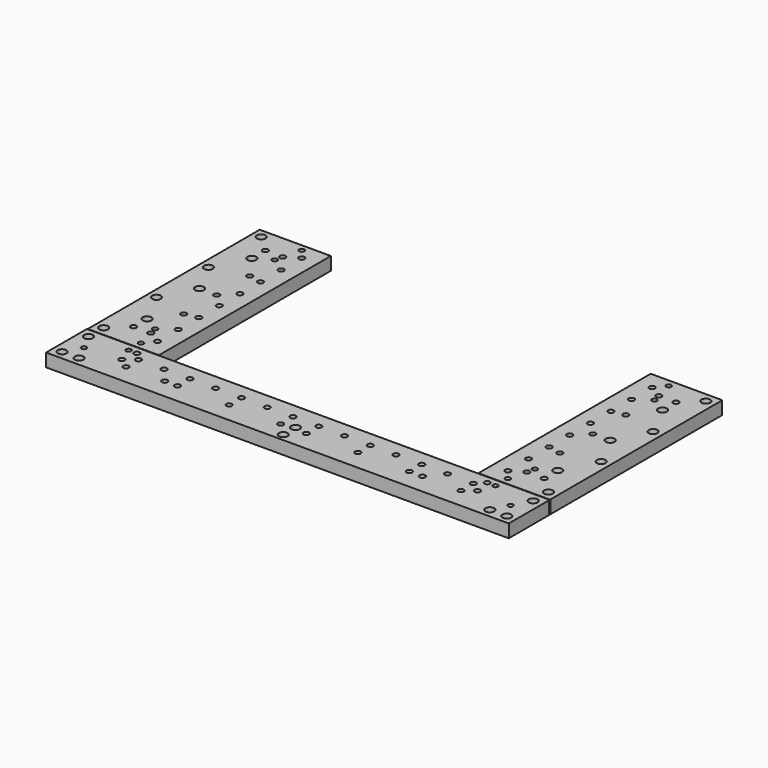
from build123d import *

# Parameters (mm, degrees)
F1_DEPTH = 25.4


# Not quite as in the source:
# - ends of sketch curves that miss each other by under 0.0002 mm in the source are joined


with BuildPart() as f1:
    # F0 (on Top) → F1 (new body)
    with BuildSketch(Plane.XY):
        Polygon((-339.0000078, 258.5000164), (-448.0000184, 258.5000164), (-448.0000184, -157.4999898), (-448.0000184, -158.4999878), (-339.414231, -158.4999878), (-310.000015, -158.4999878), (-310.000015, -157.9999888), (-310.000015, -157.4999898), (-310.000015, 258.5000164), (-310.500014, 258.5000164), align=None)
        with BuildLine():
            ThreePointArc((-431.500026, -149.0000068), (-440.0000344, -140.4999984), (-431.500026, -131.99999))
            ThreePointArc((-431.500026, -131.99999), (-423.0000176, -140.4999984), (-431.500026, -149.0000068))
        make_face(mode=Mode.SUBTRACT)
        with BuildLine():
            ThreePointArc((-356.0000246, -149.4999804), (-361.0000146, -144.4999904), (-356.0000246, -139.5000004))
            ThreePointArc((-356.0000246, -139.5000004), (-351.0000346, -144.4999904), (-356.0000246, -149.4999804))
        make_face(mode=Mode.SUBTRACT)
        with BuildLine():
            ThreePointArc((-398.5000158, -114.9999732), (-404.0000048, -109.4999842), (-398.5000158, -103.9999952))
            ThreePointArc((-398.5000158, -103.9999952), (-393.0000268, -109.4999842), (-398.5000158, -114.9999732))
        make_face(mode=Mode.SUBTRACT)
        with BuildLine():
            ThreePointArc((-340.0000058, -129.999994), (-345.4999948, -124.500005), (-340.0000058, -119.000016))
            ThreePointArc((-340.0000058, -119.000016), (-334.5000168, -124.500005), (-340.0000058, -129.999994))
        make_face(mode=Mode.SUBTRACT)
        with BuildLine():
            ThreePointArc((-365.0000066, -114.9999732), (-370.4999956, -109.4999842), (-365.0000066, -103.9999952))
            ThreePointArc((-365.0000066, -103.9999952), (-359.5000176, -109.4999842), (-365.0000066, -114.9999732))
        make_face(mode=Mode.SUBTRACT)
        with BuildLine():
            ThreePointArc((-398.5000158, -85.0000078), (-407.0000242, -76.4999994), (-398.5000158, -67.999991))
            ThreePointArc((-398.5000158, -67.999991), (-390.0000074, -76.4999994), (-398.5000158, -85.0000078))
        make_face(mode=Mode.SUBTRACT)
        with BuildLine():
            ThreePointArc((-368.500025, -99.4999788), (-373.500015, -94.4999888), (-368.500025, -89.4999988))
            ThreePointArc((-368.500025, -89.4999988), (-363.500035, -94.4999888), (-368.500025, -99.4999788))
        make_face(mode=Mode.SUBTRACT)
        with BuildLine():
            ThreePointArc((-340.0000058, -79.9999924), (-345.4999948, -74.5000034), (-340.0000058, -69.0000144))
            ThreePointArc((-340.0000058, -69.0000144), (-334.5000168, -74.5000034), (-340.0000058, -79.9999924))
        make_face(mode=Mode.SUBTRACT)
        with BuildLine():
            ThreePointArc((-431.500026, -21.0000088), (-440.0000344, -12.5000004), (-431.500026, -3.999992))
            ThreePointArc((-431.500026, -3.999992), (-423.0000176, -12.5000004), (-431.500026, -21.0000088))
        make_face(mode=Mode.SUBTRACT)
        with BuildLine():
            ThreePointArc((-365.0000066, -34.9999808), (-370.4999956, -29.4999918), (-365.0000066, -24.0000028))
            ThreePointArc((-365.0000066, -24.0000028), (-359.5000176, -29.4999918), (-365.0000066, -34.9999808))
        make_face(mode=Mode.SUBTRACT)
        with BuildLine():
            ThreePointArc((-340.0000058, -29.9999908), (-345.4999948, -24.5000018), (-340.0000058, -19.0000128))
            ThreePointArc((-340.0000058, -19.0000128), (-334.5000168, -24.5000018), (-340.0000058, -29.9999908))
        make_face(mode=Mode.SUBTRACT)
        with BuildLine():
            ThreePointArc((-340.0000058, 20.0000108), (-345.4999948, 25.4999998), (-340.0000058, 30.9999888))
            ThreePointArc((-340.0000058, 30.9999888), (-334.5000168, 25.4999998), (-340.0000058, 20.0000108))
        make_face(mode=Mode.SUBTRACT)
        with BuildLine():
            ThreePointArc((-398.5000158, 41.9999922), (-407.0000242, 50.5000006), (-398.5000158, 59.000009))
            ThreePointArc((-398.5000158, 59.000009), (-390.0000074, 50.5000006), (-398.5000158, 41.9999922))
        make_face(mode=Mode.SUBTRACT)
        with BuildLine():
            ThreePointArc((-365.0000066, 45.0000116), (-370.4999956, 50.5000006), (-365.0000066, 55.9999896))
            ThreePointArc((-365.0000066, 55.9999896), (-359.5000176, 50.5000006), (-365.0000066, 45.0000116))
        make_face(mode=Mode.SUBTRACT)
        with BuildLine():
            ThreePointArc((-340.0000058, 70.0000124), (-345.4999948, 75.5000014), (-340.0000058, 80.9999904))
            ThreePointArc((-340.0000058, 80.9999904), (-334.5000168, 75.5000014), (-340.0000058, 70.0000124))
        make_face(mode=Mode.SUBTRACT)
        with BuildLine():
            ThreePointArc((-431.500026, 104.9999932), (-440.0000344, 113.5000016), (-431.500026, 122.00001))
            ThreePointArc((-431.500026, 122.00001), (-423.0000176, 113.5000016), (-431.500026, 104.9999932))
        make_face(mode=Mode.SUBTRACT)
        with BuildLine():
            ThreePointArc((-340.0000058, 120.000014), (-345.4999948, 125.500003), (-340.0000058, 130.999992))
            ThreePointArc((-340.0000058, 130.999992), (-334.5000168, 125.500003), (-340.0000058, 120.000014))
        make_face(mode=Mode.SUBTRACT)
        with BuildLine():
            ThreePointArc((-365.0000066, 125.0000294), (-370.4999956, 130.5000184), (-365.0000066, 136.0000074))
            ThreePointArc((-365.0000066, 136.0000074), (-359.5000176, 130.5000184), (-365.0000066, 125.0000294))
        make_face(mode=Mode.SUBTRACT)
        with BuildLine():
            ThreePointArc((-398.5000158, 168.9999922), (-407.0000242, 177.5000006), (-398.5000158, 186.000009))
            ThreePointArc((-398.5000158, 186.000009), (-390.0000074, 177.5000006), (-398.5000158, 168.9999922))
        make_face(mode=Mode.SUBTRACT)
        with BuildLine():
            ThreePointArc((-340.0000058, 170.0000156), (-345.4999948, 175.5000046), (-340.0000058, 180.9999936))
            ThreePointArc((-340.0000058, 180.9999936), (-334.5000168, 175.5000046), (-340.0000058, 170.0000156))
        make_face(mode=Mode.SUBTRACT)
        with BuildLine():
            ThreePointArc((-398.5000158, 205.0000218), (-404.0000048, 210.5000108), (-398.5000158, 215.9999998))
            ThreePointArc((-398.5000158, 215.9999998), (-393.0000268, 210.5000108), (-398.5000158, 205.0000218))
        make_face(mode=Mode.SUBTRACT)
        with BuildLine():
            ThreePointArc((-368.500025, 190.5000254), (-373.500015, 195.5000154), (-368.500025, 200.5000054))
            ThreePointArc((-368.500025, 200.5000054), (-363.500035, 195.5000154), (-368.500025, 190.5000254))
        make_face(mode=Mode.SUBTRACT)
        with BuildLine():
            ThreePointArc((-365.0000066, 205.0000218), (-370.4999956, 210.5000108), (-365.0000066, 215.9999998))
            ThreePointArc((-365.0000066, 215.9999998), (-359.5000176, 210.5000108), (-365.0000066, 205.0000218))
        make_face(mode=Mode.SUBTRACT)
        with BuildLine():
            ThreePointArc((-340.0000058, 220.0000172), (-345.4999948, 225.5000062), (-340.0000058, 230.9999952))
            ThreePointArc((-340.0000058, 230.9999952), (-334.5000168, 225.5000062), (-340.0000058, 220.0000172))
        make_face(mode=Mode.SUBTRACT)
        with BuildLine():
            ThreePointArc((-431.500026, 232.9999912), (-440.0000344, 241.4999996), (-431.500026, 250.000008))
            ThreePointArc((-431.500026, 250.000008), (-423.0000176, 241.4999996), (-431.500026, 232.9999912))
        make_face(mode=Mode.SUBTRACT)
        with BuildLine():
            ThreePointArc((-356.0000246, 240.500027), (-361.0000146, 245.500017), (-356.0000246, 250.500007))
            ThreePointArc((-356.0000246, 250.500007), (-351.0000346, 245.500017), (-356.0000246, 240.500027))
        make_face(mode=Mode.SUBTRACT)
    extrude(amount=F1_DEPTH)


with BuildPart() as f1b:
    # F0 (on Top) → F1, piece 2 (new body)
    with BuildSketch(Plane.XY):
        Polygon((-448.0000184, -258.499991), (-333.0000198, -258.499991), (-65.0000224, -258.499991), (64.9999716, -258.499991), (332.9999944, -258.499991), (447.999993, -258.499991), (448.999991, -258.499991), (448.999991, -160.4999838), (448.499992, -159.9999848), (447.999993, -159.4999858), (332.9999944, -159.4999858), (-333.0000198, -159.4999858), (-448.0000184, -159.4999858), (-448.2500179, -159.7499853), (-448.5000174, -159.9999848), (-449.0000164, -160.4999838), (-449.0000164, -258.499991), align=None)
        with BuildLine():
            ThreePointArc((-423.0000176, -241.4999996), (-431.500026, -250.000008), (-440.0000344, -241.4999996))
            ThreePointArc((-440.0000344, -241.4999996), (-431.500026, -232.9999912), (-423.0000176, -241.4999996))
        make_face(mode=Mode.SUBTRACT)
        with BuildLine():
            ThreePointArc((-390.0000074, -241.4999996), (-398.5000158, -250.000008), (-407.0000242, -241.4999996))
            ThreePointArc((-407.0000242, -241.4999996), (-398.5000158, -232.9999912), (-390.0000074, -241.4999996))
        make_face(mode=Mode.SUBTRACT)
        with BuildLine():
            ThreePointArc((-409.0000202, -210.4999854), (-414.0000102, -215.4999754), (-419.0000002, -210.4999854))
            ThreePointArc((-419.0000002, -210.4999854), (-414.0000102, -205.4999954), (-409.0000202, -210.4999854))
        make_face(mode=Mode.SUBTRACT)
        with BuildLine():
            ThreePointArc((-339.5000322, -204.4999974), (-345.0000212, -209.9999864), (-350.5000102, -204.4999974))
            ThreePointArc((-350.5000102, -204.4999974), (-345.0000212, -199.0000084), (-339.5000322, -204.4999974))
        make_face(mode=Mode.SUBTRACT)
        with BuildLine():
            ThreePointArc((-319.5000214, -219.4999928), (-325.0000104, -224.9999818), (-330.4999994, -219.4999928))
            ThreePointArc((-330.4999994, -219.4999928), (-325.0000104, -214.0000038), (-319.5000214, -219.4999928))
        make_face(mode=Mode.SUBTRACT)
        with BuildLine():
            ThreePointArc((-244.500019, -219.4999928), (-250.000008, -224.9999818), (-255.499997, -219.4999928))
            ThreePointArc((-255.499997, -219.4999928), (-250.000008, -214.0000038), (-244.500019, -219.4999928))
        make_face(mode=Mode.SUBTRACT)
        with BuildLine():
            ThreePointArc((-219.5000182, -219.4999928), (-225.0000072, -224.9999818), (-230.4999962, -219.4999928))
            ThreePointArc((-230.4999962, -219.4999928), (-225.0000072, -214.0000038), (-219.5000182, -219.4999928))
        make_face(mode=Mode.SUBTRACT)
        with BuildLine():
            ThreePointArc((-423.0000176, -177.5000006), (-431.500026, -186.000009), (-440.0000344, -177.5000006))
            ThreePointArc((-440.0000344, -177.5000006), (-431.500026, -168.9999922), (-423.0000176, -177.5000006))
        make_face(mode=Mode.SUBTRACT)
        with BuildLine():
            ThreePointArc((-351.0000346, -174.4999812), (-356.0000246, -179.4999712), (-361.0000146, -174.4999812))
            ThreePointArc((-361.0000146, -174.4999812), (-356.0000246, -169.4999912), (-351.0000346, -174.4999812))
        make_face(mode=Mode.SUBTRACT)
        with BuildLine():
            ThreePointArc((-334.5000168, -174.4999812), (-340.0000058, -179.9999702), (-345.4999948, -174.4999812))
            ThreePointArc((-345.4999948, -174.4999812), (-340.0000058, -168.9999922), (-334.5000168, -174.4999812))
        make_face(mode=Mode.SUBTRACT)
        with BuildLine():
            ThreePointArc((-319.5000214, -189.500002), (-325.0000104, -194.999991), (-330.4999994, -189.500002))
            ThreePointArc((-330.4999994, -189.500002), (-325.0000104, -184.000013), (-319.5000214, -189.500002))
        make_face(mode=Mode.SUBTRACT)
        with BuildLine():
            ThreePointArc((-269.5000198, -189.500002), (-275.0000088, -194.999991), (-280.4999978, -189.500002))
            ThreePointArc((-280.4999978, -189.500002), (-275.0000088, -184.000013), (-269.5000198, -189.500002))
        make_face(mode=Mode.SUBTRACT)
        with BuildLine():
            ThreePointArc((-219.5000182, -189.500002), (-225.0000072, -194.999991), (-230.4999962, -189.500002))
            ThreePointArc((-230.4999962, -189.500002), (-225.0000072, -184.000013), (-219.5000182, -189.500002))
        make_face(mode=Mode.SUBTRACT)
        with BuildLine():
            ThreePointArc((-119.500015, -219.4999928), (-125.000004, -224.9999818), (-130.499993, -219.4999928))
            ThreePointArc((-130.499993, -219.4999928), (-125.000004, -214.0000038), (-119.500015, -219.4999928))
        make_face(mode=Mode.SUBTRACT)
        with BuildLine():
            ThreePointArc((8.499983, -244.4999936), (-2.54e-05, -253.000002), (-8.5000338, -244.4999936))
            ThreePointArc((-8.5000338, -244.4999936), (-2.54e-05, -235.9999852), (8.499983, -244.4999936))
        make_face(mode=Mode.SUBTRACT)
        with BuildLine():
            ThreePointArc((-19.5000372, -219.4999928), (-25.0000262, -224.9999818), (-30.5000152, -219.4999928))
            ThreePointArc((-30.5000152, -219.4999928), (-25.0000262, -214.0000038), (-19.5000372, -219.4999928))
        make_face(mode=Mode.SUBTRACT)
        with BuildLine():
            ThreePointArc((8.499983, -214.5000028), (-2.54e-05, -223.0000112), (-8.5000338, -214.5000028))
            ThreePointArc((-8.5000338, -214.5000028), (-2.54e-05, -205.9999944), (8.499983, -214.5000028))
        make_face(mode=Mode.SUBTRACT)
        with BuildLine():
            ThreePointArc((-169.5000166, -189.500002), (-175.0000056, -194.999991), (-180.4999946, -189.500002))
            ThreePointArc((-180.4999946, -189.500002), (-175.0000056, -184.000013), (-169.5000166, -189.500002))
        make_face(mode=Mode.SUBTRACT)
        with BuildLine():
            ThreePointArc((-119.500015, -189.500002), (-125.000004, -194.999991), (-130.499993, -189.500002))
            ThreePointArc((-130.499993, -189.500002), (-125.000004, -184.000013), (-119.500015, -189.500002))
        make_face(mode=Mode.SUBTRACT)
        with BuildLine():
            ThreePointArc((-69.5000388, -189.500002), (-75.0000278, -194.999991), (-80.5000168, -189.500002))
            ThreePointArc((-80.5000168, -189.500002), (-75.0000278, -184.000013), (-69.5000388, -189.500002))
        make_face(mode=Mode.SUBTRACT)
        with BuildLine():
            ThreePointArc((-19.5000372, -189.500002), (-25.0000262, -194.999991), (-30.5000152, -189.500002))
            ThreePointArc((-30.5000152, -189.500002), (-25.0000262, -184.000013), (-19.5000372, -189.500002))
        make_face(mode=Mode.SUBTRACT)
        with BuildLine():
            ThreePointArc((30.4999644, -219.4999928), (24.9999754, -224.9999818), (19.4999864, -219.4999928))
            ThreePointArc((19.4999864, -219.4999928), (24.9999754, -214.0000038), (30.4999644, -219.4999928))
        make_face(mode=Mode.SUBTRACT)
        with BuildLine():
            ThreePointArc((130.4999676, -219.4999928), (124.9999786, -224.9999818), (119.4999896, -219.4999928))
            ThreePointArc((119.4999896, -219.4999928), (124.9999786, -214.0000038), (130.4999676, -219.4999928))
        make_face(mode=Mode.SUBTRACT)
        with BuildLine():
            ThreePointArc((30.4999644, -189.500002), (24.9999754, -194.999991), (19.4999864, -189.500002))
            ThreePointArc((19.4999864, -189.500002), (24.9999754, -184.000013), (30.4999644, -189.500002))
        make_face(mode=Mode.SUBTRACT)
        with BuildLine():
            ThreePointArc((80.499966, -189.500002), (74.999977, -194.999991), (69.499988, -189.500002))
            ThreePointArc((69.499988, -189.500002), (74.999977, -184.000013), (80.499966, -189.500002))
        make_face(mode=Mode.SUBTRACT)
        with BuildLine():
            ThreePointArc((130.4999676, -189.500002), (124.9999786, -194.999991), (119.4999896, -189.500002))
            ThreePointArc((119.4999896, -189.500002), (124.9999786, -184.000013), (130.4999676, -189.500002))
        make_face(mode=Mode.SUBTRACT)
        with BuildLine():
            ThreePointArc((180.4999692, -189.500002), (174.9999802, -194.999991), (169.4999912, -189.500002))
            ThreePointArc((169.4999912, -189.500002), (174.9999802, -184.000013), (180.4999692, -189.500002))
        make_face(mode=Mode.SUBTRACT)
        with BuildLine():
            ThreePointArc((230.4999708, -219.4999928), (224.9999818, -224.9999818), (219.4999928, -219.4999928))
            ThreePointArc((219.4999928, -219.4999928), (224.9999818, -214.0000038), (230.4999708, -219.4999928))
        make_face(mode=Mode.SUBTRACT)
        with BuildLine():
            ThreePointArc((255.4999716, -219.4999928), (249.9999826, -224.9999818), (244.4999936, -219.4999928))
            ThreePointArc((244.4999936, -219.4999928), (249.9999826, -214.0000038), (255.4999716, -219.4999928))
        make_face(mode=Mode.SUBTRACT)
        with BuildLine():
            ThreePointArc((330.499974, -219.4999928), (324.999985, -224.9999818), (319.499996, -219.4999928))
            ThreePointArc((319.499996, -219.4999928), (324.999985, -214.0000038), (330.499974, -219.4999928))
        make_face(mode=Mode.SUBTRACT)
        with BuildLine():
            ThreePointArc((406.9999988, -241.4999996), (398.4999904, -250.000008), (389.999982, -241.4999996))
            ThreePointArc((389.999982, -241.4999996), (398.4999904, -232.9999912), (406.9999988, -241.4999996))
        make_face(mode=Mode.SUBTRACT)
        with BuildLine():
            ThreePointArc((439.9999836, -241.4999996), (431.4999752, -250.000008), (422.9999668, -241.4999996))
            ThreePointArc((422.9999668, -241.4999996), (431.4999752, -232.9999912), (439.9999836, -241.4999996))
        make_face(mode=Mode.SUBTRACT)
        with BuildLine():
            ThreePointArc((350.4999848, -204.4999974), (344.9999958, -209.9999864), (339.5000068, -204.4999974))
            ThreePointArc((339.5000068, -204.4999974), (344.9999958, -199.0000084), (350.4999848, -204.4999974))
        make_face(mode=Mode.SUBTRACT)
        with BuildLine():
            ThreePointArc((418.9999748, -210.4999854), (413.9999848, -215.4999754), (408.9999948, -210.4999854))
            ThreePointArc((408.9999948, -210.4999854), (413.9999848, -205.4999954), (418.9999748, -210.4999854))
        make_face(mode=Mode.SUBTRACT)
        with BuildLine():
            ThreePointArc((230.4999708, -189.500002), (224.9999818, -194.999991), (219.4999928, -189.500002))
            ThreePointArc((219.4999928, -189.500002), (224.9999818, -184.000013), (230.4999708, -189.500002))
        make_face(mode=Mode.SUBTRACT)
        with BuildLine():
            ThreePointArc((280.4999724, -189.500002), (274.9999834, -194.999991), (269.4999944, -189.500002))
            ThreePointArc((269.4999944, -189.500002), (274.9999834, -184.000013), (280.4999724, -189.500002))
        make_face(mode=Mode.SUBTRACT)
        with BuildLine():
            ThreePointArc((330.499974, -189.500002), (324.999985, -194.999991), (319.499996, -189.500002))
            ThreePointArc((319.499996, -189.500002), (324.999985, -184.000013), (330.499974, -189.500002))
        make_face(mode=Mode.SUBTRACT)
        with BuildLine():
            ThreePointArc((345.4999694, -174.4999812), (339.9999804, -179.9999702), (334.4999914, -174.4999812))
            ThreePointArc((334.4999914, -174.4999812), (339.9999804, -168.9999922), (345.4999694, -174.4999812))
        make_face(mode=Mode.SUBTRACT)
        with BuildLine():
            ThreePointArc((360.9999638, -174.4999812), (355.9999738, -179.4999712), (350.9999838, -174.4999812))
            ThreePointArc((350.9999838, -174.4999812), (355.9999738, -169.4999912), (360.9999638, -174.4999812))
        make_face(mode=Mode.SUBTRACT)
        with BuildLine():
            ThreePointArc((439.9999836, -177.5000006), (431.4999752, -186.000009), (422.9999668, -177.5000006))
            ThreePointArc((422.9999668, -177.5000006), (431.4999752, -168.9999922), (439.9999836, -177.5000006))
        make_face(mode=Mode.SUBTRACT)
    extrude(amount=F1_DEPTH)


with BuildPart() as f1c:
    # F0 (on Top) → F1, piece 3 (new body)
    with BuildSketch(Plane.XY):
        Polygon((309.9999896, 258.5000164), (309.9999896, -157.4999898), (309.9999896, -157.9999888), (309.9999896, -158.4999878), (339.4142056, -158.4999878), (447.999993, -158.4999878), (448.499992, -157.9999888), (448.999991, -157.4999898), (448.999991, 258.5000164), (448.499992, 259.0000154), (447.999993, 259.5000144), (339.4142056, 259.5000144), (309.9999896, 259.5000144), (309.9999896, 259.0000154), (310.4999886, 258.5000164), align=None)
        with BuildLine():
            ThreePointArc((355.9999738, -139.5000004), (360.9999638, -144.4999904), (355.9999738, -149.4999804))
            ThreePointArc((355.9999738, -149.4999804), (350.9999838, -144.4999904), (355.9999738, -139.5000004))
        make_face(mode=Mode.SUBTRACT)
        with BuildLine():
            ThreePointArc((431.4999752, -131.99999), (439.9999836, -140.4999984), (431.4999752, -149.0000068))
            ThreePointArc((431.4999752, -149.0000068), (422.9999668, -140.4999984), (431.4999752, -131.99999))
        make_face(mode=Mode.SUBTRACT)
        with BuildLine():
            ThreePointArc((339.9999804, -119.000016), (345.4999694, -124.500005), (339.9999804, -129.999994))
            ThreePointArc((339.9999804, -129.999994), (334.4999914, -124.500005), (339.9999804, -119.000016))
        make_face(mode=Mode.SUBTRACT)
        with BuildLine():
            ThreePointArc((364.9999812, -103.9999952), (370.4999702, -109.4999842), (364.9999812, -114.9999732))
            ThreePointArc((364.9999812, -114.9999732), (359.4999922, -109.4999842), (364.9999812, -103.9999952))
        make_face(mode=Mode.SUBTRACT)
        with BuildLine():
            ThreePointArc((398.4999904, -103.9999952), (403.9999794, -109.4999842), (398.4999904, -114.9999732))
            ThreePointArc((398.4999904, -114.9999732), (393.0000014, -109.4999842), (398.4999904, -103.9999952))
        make_face(mode=Mode.SUBTRACT)
        with BuildLine():
            ThreePointArc((368.4999742, -89.4999988), (373.4999642, -94.4999888), (368.4999742, -99.4999788))
            ThreePointArc((368.4999742, -99.4999788), (363.4999842, -94.4999888), (368.4999742, -89.4999988))
        make_face(mode=Mode.SUBTRACT)
        with BuildLine():
            ThreePointArc((339.9999804, -69.0000144), (345.4999694, -74.5000034), (339.9999804, -79.9999924))
            ThreePointArc((339.9999804, -79.9999924), (334.4999914, -74.5000034), (339.9999804, -69.0000144))
        make_face(mode=Mode.SUBTRACT)
        with BuildLine():
            ThreePointArc((398.4999904, -67.999991), (406.9999988, -76.4999994), (398.4999904, -85.0000078))
            ThreePointArc((398.4999904, -85.0000078), (389.999982, -76.4999994), (398.4999904, -67.999991))
        make_face(mode=Mode.SUBTRACT)
        with BuildLine():
            ThreePointArc((339.9999804, -19.0000128), (345.4999694, -24.5000018), (339.9999804, -29.9999908))
            ThreePointArc((339.9999804, -29.9999908), (334.4999914, -24.5000018), (339.9999804, -19.0000128))
        make_face(mode=Mode.SUBTRACT)
        with BuildLine():
            ThreePointArc((364.9999812, -24.0000028), (370.4999702, -29.4999918), (364.9999812, -34.9999808))
            ThreePointArc((364.9999812, -34.9999808), (359.4999922, -29.4999918), (364.9999812, -24.0000028))
        make_face(mode=Mode.SUBTRACT)
        with BuildLine():
            ThreePointArc((431.4999752, -3.999992), (439.9999836, -12.5000004), (431.4999752, -21.0000088))
            ThreePointArc((431.4999752, -21.0000088), (422.9999668, -12.5000004), (431.4999752, -3.999992))
        make_face(mode=Mode.SUBTRACT)
        with BuildLine():
            ThreePointArc((339.9999804, 30.9999888), (345.4999694, 25.4999998), (339.9999804, 20.0000108))
            ThreePointArc((339.9999804, 20.0000108), (334.4999914, 25.4999998), (339.9999804, 30.9999888))
        make_face(mode=Mode.SUBTRACT)
        with BuildLine():
            ThreePointArc((364.9999812, 55.9999896), (370.4999702, 50.5000006), (364.9999812, 45.0000116))
            ThreePointArc((364.9999812, 45.0000116), (359.4999922, 50.5000006), (364.9999812, 55.9999896))
        make_face(mode=Mode.SUBTRACT)
        with BuildLine():
            ThreePointArc((398.4999904, 59.000009), (406.9999988, 50.5000006), (398.4999904, 41.9999922))
            ThreePointArc((398.4999904, 41.9999922), (389.999982, 50.5000006), (398.4999904, 59.000009))
        make_face(mode=Mode.SUBTRACT)
        with BuildLine():
            ThreePointArc((339.9999804, 80.9999904), (345.4999694, 75.5000014), (339.9999804, 70.0000124))
            ThreePointArc((339.9999804, 70.0000124), (334.4999914, 75.5000014), (339.9999804, 80.9999904))
        make_face(mode=Mode.SUBTRACT)
        with BuildLine():
            ThreePointArc((339.9999804, 130.999992), (345.4999694, 125.500003), (339.9999804, 120.000014))
            ThreePointArc((339.9999804, 120.000014), (334.4999914, 125.500003), (339.9999804, 130.999992))
        make_face(mode=Mode.SUBTRACT)
        with BuildLine():
            ThreePointArc((431.4999752, 122.00001), (439.9999836, 113.5000016), (431.4999752, 104.9999932))
            ThreePointArc((431.4999752, 104.9999932), (422.9999668, 113.5000016), (431.4999752, 122.00001))
        make_face(mode=Mode.SUBTRACT)
        with BuildLine():
            ThreePointArc((364.9999812, 136.0000074), (370.4999702, 130.5000184), (364.9999812, 125.0000294))
            ThreePointArc((364.9999812, 125.0000294), (359.4999922, 130.5000184), (364.9999812, 136.0000074))
        make_face(mode=Mode.SUBTRACT)
        with BuildLine():
            ThreePointArc((339.9999804, 180.9999936), (345.4999694, 175.5000046), (339.9999804, 170.0000156))
            ThreePointArc((339.9999804, 170.0000156), (334.4999914, 175.5000046), (339.9999804, 180.9999936))
        make_face(mode=Mode.SUBTRACT)
        with BuildLine():
            ThreePointArc((398.4999904, 186.000009), (406.9999988, 177.5000006), (398.4999904, 168.9999922))
            ThreePointArc((398.4999904, 168.9999922), (389.999982, 177.5000006), (398.4999904, 186.000009))
        make_face(mode=Mode.SUBTRACT)
        with BuildLine():
            ThreePointArc((368.4999742, 200.5000054), (373.4999642, 195.5000154), (368.4999742, 190.5000254))
            ThreePointArc((368.4999742, 190.5000254), (363.4999842, 195.5000154), (368.4999742, 200.5000054))
        make_face(mode=Mode.SUBTRACT)
        with BuildLine():
            ThreePointArc((364.9999812, 215.9999998), (370.4999702, 210.5000108), (364.9999812, 205.0000218))
            ThreePointArc((364.9999812, 205.0000218), (359.4999922, 210.5000108), (364.9999812, 215.9999998))
        make_face(mode=Mode.SUBTRACT)
        with BuildLine():
            ThreePointArc((339.9999804, 230.9999952), (345.4999694, 225.5000062), (339.9999804, 220.0000172))
            ThreePointArc((339.9999804, 220.0000172), (334.4999914, 225.5000062), (339.9999804, 230.9999952))
        make_face(mode=Mode.SUBTRACT)
        with BuildLine():
            ThreePointArc((398.4999904, 215.9999998), (403.9999794, 210.5000108), (398.4999904, 205.0000218))
            ThreePointArc((398.4999904, 205.0000218), (393.0000014, 210.5000108), (398.4999904, 215.9999998))
        make_face(mode=Mode.SUBTRACT)
        with BuildLine():
            ThreePointArc((355.9999738, 250.500007), (360.9999638, 245.500017), (355.9999738, 240.500027))
            ThreePointArc((355.9999738, 240.500027), (350.9999838, 245.500017), (355.9999738, 250.500007))
        make_face(mode=Mode.SUBTRACT)
        with BuildLine():
            ThreePointArc((431.4999752, 250.000008), (439.9999836, 241.4999996), (431.4999752, 232.9999912))
            ThreePointArc((431.4999752, 232.9999912), (422.9999668, 241.4999996), (431.4999752, 250.000008))
        make_face(mode=Mode.SUBTRACT)
    extrude(amount=F1_DEPTH)


solid = Compound([f1.part, f1b.part, f1c.part])
